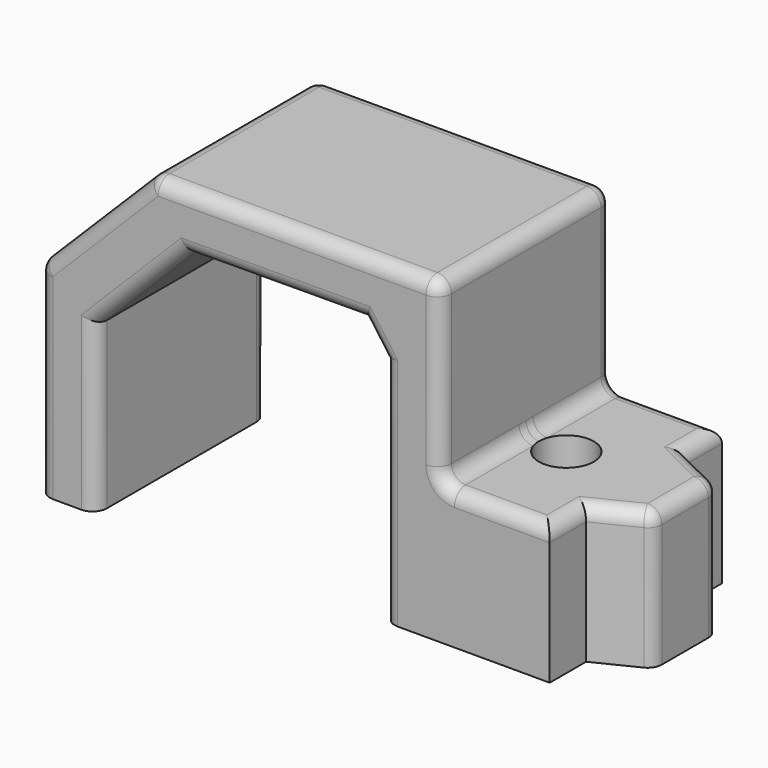
from build123d import *

# Parameters (mm, degrees)
F1_DEPTH = 9.6266
F3_D     = 2.4638
F5_DEPTH = 6.1449664227
F6_R     = 0.635


# Not quite as in the source:
# - a feature names something its author has since deleted; it is built from what else it names


with BuildPart() as f1:
    # F0 (on Front) → F1 (new body)
    with BuildSketch(Plane.XZ):
        Polygon((-7.4422, 0), (0, 0), (0, 6.1449664227), (-4.9022, 6.1449664227), (-4.9022, 14.097), (-17.78, 14.097), (-22.86, 9.017), (-22.86, 0), (-20.32, 0), (-20.32, 7.4086618234), (-16.2178584248, 11.5251476239), (-8.3548940885, 11.5611667216), (-7.4422, 10.294130072), align=None)
    extrude(amount=F1_DEPTH)

    # F3 (through all)
    with Locations(Plane(origin=(0, 0, 0), x_dir=(1, 0, 0), z_dir=(0, 0, -1))):
        with Locations((-3.0988, 4.826)):
            Hole(F3_D / 2)

    # F4 (on Top) → F5 (join, through all)
    with BuildSketch(Plane.XY):
        Polygon((0, -2.032), (0, -7.5946), (2.2016586276, -6.5053654334), (2.2016586276, -3.1212345666), align=None)
    extrude(amount=F5_DEPTH)

    # F6
    f6_edges = [f1.edges().sort_by_distance(p)[0] for p in [
        (-7.4422, 0, 5.147065),
        (-7.898547, 0, 10.927648),
        (-12.286376, 0, 11.543157),
        (-20.32, 0, 3.704331),
        (-20.32, -9.6266, 3.704331),
        (-12.286376, -9.6266, 11.543157),
        (-7.898547, -9.6266, 10.927648),
        (-7.4422, -9.6266, 5.147065),
        (-4.9022, 0, 10.120983),
        (-4.9022, -9.6266, 10.120983),
        (0, -1.016, 6.144966),
        (0, -8.6106, 6.144966),
        (-2.4511, 0, 6.144966),
        (-2.4511, -9.6266, 6.144966),
        (-20.32, -9.6266, 11.557),
        (-22.86, -9.6266, 4.5085),
        (-18.268929, -9.6266, 9.466905),
        (-20.32, 0, 11.557),
        (-22.86, 0, 4.5085),
        (-18.268929, 0, 9.466905),
        (-11.3411, 0, 14.097),
        (-11.3411, -9.6266, 14.097),
        (-17.78, -4.8133, 14.097),
        (-22.86, -4.8133, 9.017),
        (1.100829, -7.049983, 6.144966),
        (2.201659, -4.8133, 6.144966),
        (1.100829, -2.576617, 6.144966),
        (2.201659, -6.505365, 3.072483),
        (2.201659, -3.121235, 3.072483),
        (-4.9022, -4.8133, 6.144966),
        (-4.9022, -4.8133, 14.097),
    ]]
    fillet(f6_edges, radius=F6_R)


solid = f1.part
